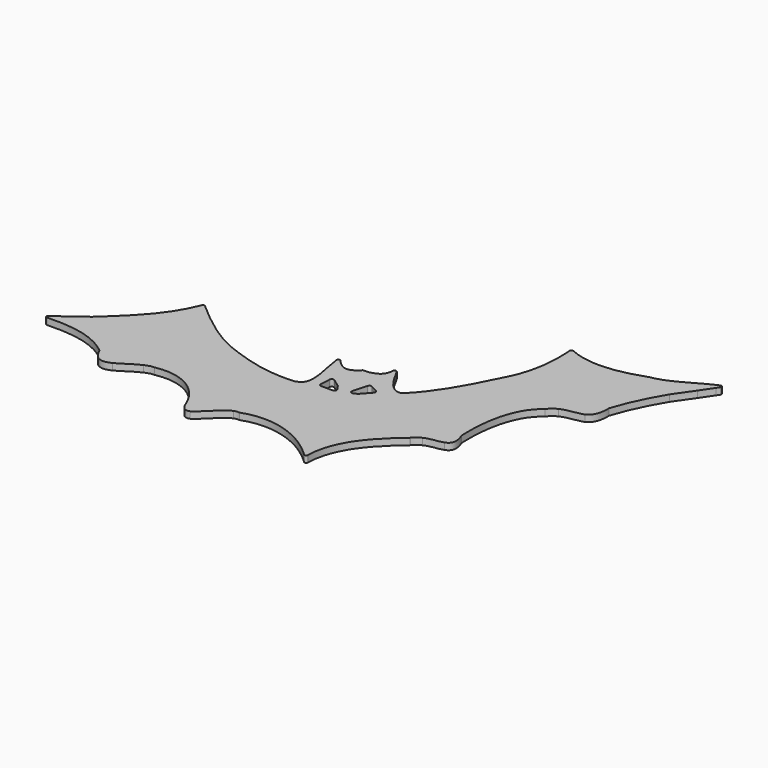
from build123d import *

# Parameters (mm, degrees)
F1_DEPTH    = 1.2
F2_R        = 0.3
F3_T1_DEPTH = 1.2
F4_R        = 0.4


# Not quite as in the source:
# - a fillet or chamfer that OpenCascade refuses, or shapes differently, is made with other operations: its cross-section is extruded or revolved along the edge and cut away or added


with BuildPart() as f1:
    # F0 (on Top) → F1 (new body)
    with BuildSketch(Plane.XY):
        with BuildLine():
            add(Edge.make_bspline(
                [(-38.4798780204, -12.2663156816), (-39.544490026, -13.1099494205), (-40.6234752996, -13.9226719378), (-41.7197013285, -14.6909028127)],
                knots=[0, 0, 0, 0, 0.5352911652, 0.5352911652, 0.5352911652, 0.5352911652], degree=3))
            add(Edge.make_bspline(
                [(-41.7197013286, -14.6909028123), (-38.0795273857, -14.7004525366), (-34.4057833476, -15.3318172874), (-31.2715117029, -17.7636174939)],
                knots=[0.2133521121, 0.2133521121, 0.2133521121, 0.2133521121, 1, 1, 1, 1], degree=3))
            add(Edge.make_bspline(
                [(-31.2715117029, -17.7636174939), (-29.0153017657, -22.7858694917), (-25.5082486685, -17.0450166263), (-22.2937322686, -17.0941546532)],
                knots=[0, 0, 0, 0, 1, 1, 1, 1], degree=3))
            add(Edge.make_bspline(
                [(-22.2937322686, -17.0941546532), (-18.3303199267, -16.3920818703), (-14.1754137574, -17.8912452003), (-12.0371793955, -22.4632093461)],
                knots=[0, 0, 0, 0, 1, 1, 1, 1], degree=3))
            add(Edge.make_bspline(
                [(-12.0371793955, -22.4632093461), (-10.273242702, -27.2684784847), (-7.0541938207, -19.6953683351), (-4.1345165041, -20.0729846223)],
                knots=[0, 0, 0, 0, 1, 1, 1, 1], degree=3))
            add(Edge.make_bspline(
                [(-4.1345165041, -20.0729846223), (1.2434419273, -18.2527364634), (7.1570299201, -20.3861330581), (11.4834791975, -24.5899863856)],
                knots=[0, 0, 0, 0, 1, 1, 1, 1], degree=3))
            add(Edge.make_bspline(
                [(11.4834791975, -24.5899863856), (11.3410479857, -18.4819489611), (15.805950917, -14.5268131434), (19.4643467655, -11.5875236785)],
                knots=[0, 0, 0, 0, 1, 1, 1, 1], degree=3))
            add(Edge.make_bspline(
                [(19.4643467655, -11.5875236785), (20.8953696781, -9.465229862), (24.9063475432, -10.9951342488), (24.8114189767, -8.5803924237)],
                knots=[0, 0, 0, 0, 0.8539890071, 0.8539890071, 0.8539890071, 0.8539890071], degree=3))
            add(Edge.make_bspline(
                [(24.8114189767, -8.5803924237), (24.7715269271, -8.4685484651), (24.7275843922, -8.3524176209), (24.6794406334, -8.2318174934)],
                knots=[0.9759440179, 0.9759440179, 0.9759440179, 0.9759440179, 1, 1, 1, 1], degree=3))
            add(Edge.make_bspline(
                [(24.6794406334, -8.2318174934), (24.6721729206, -8.0739743472), (24.6659042214, -7.915212537), (24.6606897414, -7.7556620666)],
                knots=[0, 0, 0, 0, 0.0312727725, 0.0312727725, 0.0312727725, 0.0312727725], degree=3))
            add(Edge.make_bspline(
                [(24.6606897414, -7.7556620666), (24.5901871692, -7.5161203522), (24.4939231594, -7.2512100585), (24.3692332397, -6.9579036653)],
                knots=[0.9371550745, 0.9371550745, 0.9371550745, 0.9371550745, 1, 1, 1, 1], degree=3))
            add(Edge.make_bspline(
                [(24.3692332397, -6.9579036653), (24.1388380843, -2.2591127335), (24.9211464491, 3.314156379), (28.5056438685, 5.8047525516)],
                knots=[0, 0, 0, 0, 1, 1, 1, 1], degree=3))
            add(Edge.make_bspline(
                [(28.5056438685, 5.8047525516), (30.9062919992, 8.9355748498), (35.8582398281, 5.7820329361), (35.6726384866, 11.4003236568)],
                knots=[0, 0, 0, 0, 1, 1, 1, 1], degree=3))
            add(Edge.make_bspline(
                [(35.6726384866, 11.4003236568), (36.7663971201, 14.6066645914), (38.3424158626, 17.4642666985), (40.1032277755, 20.1498568209)],
                knots=[0, 0, 0, 0, 0.5755878955, 0.5755878955, 0.5755878955, 0.5755878955], degree=3))
            add(Edge.make_bspline(
                [(40.1032277755, 20.1498568209), (41.2585835018, 22.0843550242), (42.5070626066, 23.9305479484), (43.7611872479, 25.743781902)],
                knots=[0.5268633096, 0.5268633096, 0.5268633096, 0.5268633096, 0.908526515, 0.908526515, 0.908526515, 0.908526515], degree=3))
            add(Edge.make_bspline(
                [(43.7611872479, 25.743781902), (40.5051598058, 24.6156248297), (37.6057351876, 22.1634385625), (34.1849912478, 21.6757304041)],
                knots=[0.0409615452, 0.0409615452, 0.0409615452, 0.0409615452, 1, 1, 1, 1], degree=3))
            add(Edge.make_bspline(
                [(34.1849912478, 21.6757304041), (29.819862337, 20.2040716593), (25.0759812483, 19.4382459028), (20.7234813058, 21.313829756)],
                knots=[0, 0, 0, 0, 0.9509269262, 0.9509269262, 0.9509269262, 0.9509269262], degree=3))
            add(Edge.make_bspline(
                [(20.7234813058, 21.313829756), (20.9800191175, 17.2558597069), (20.4243543566, 13.0954506221), (18.5978538652, 9.7460444081)],
                knots=[0.0959141779, 0.0959141779, 0.0959141779, 0.0959141779, 1, 1, 1, 1], degree=3))
            add(Edge.make_bspline(
                [(18.5978538652, 9.7460444081), (16.277791329, 4.965444658), (13.734376016, 0.0795420777), (10.2447861041, -3.272037287)],
                knots=[0, 0, 0, 0, 1, 1, 1, 1], degree=3))
            add(Edge.make_bspline(
                [(10.2447861041, -3.272037287), (10.1955990612, -3.2702979601), (10.1468874332, -3.2670014327), (10.0986391366, -3.2621927773)],
                knots=[0, 0, 0, 0, 0.0194783611, 0.0194783611, 0.0194783611, 0.0194783611], degree=3))
            add(Edge.make_bspline(
                [(10.0986391274, -3.2621927392), (10.0510770286, -3.3087890461), (10.0033383979, -3.3551002989), (9.9554213638, -3.4011222524)],
                knots=[0.9862685814, 0.9862685814, 0.9862685814, 0.9862685814, 1, 1, 1, 1], degree=3))
            add(Edge.make_bspline(
                [(9.9554213638, -3.4011222524), (7.6435278836, -3.319370212), (6.3819190636, 0.2025468295), (4.915882773, 2.4844337463)],
                knots=[0, 0, 0, 0, 0.9155241129, 0.9155241129, 0.9155241129, 0.9155241129], degree=3))
            add(Edge.make_bspline(
                [(4.915882772, 2.4844337459), (5.1701481527, 0.5226394908), (4.5999139224, -0.4439197046), (3.5342091981, -0.8428686021)],
                knots=[0.072121838, 0.072121838, 0.072121838, 0.072121838, 0.6923701781, 0.6923701781, 0.6923701781, 0.6923701781], degree=3))
            add(Edge.make_bspline(
                [(3.5342091981, -0.8428686021), (3.0006050925, -1.1239670726), (2.3072433966, -1.2205903145), (1.5090960129, -1.2041829107)],
                knots=[0.6335885985, 0.6335885985, 0.6335885985, 0.6335885985, 0.9752013666, 0.9752013666, 0.9752013666, 0.9752013666], degree=3))
            add(Edge.make_bspline(
                [(1.5090960151, -1.2041829145), (1.0819239999, -1.6929707802), (0.6747439774, -1.9863590245), (0.2827989549, -2.124205249)],
                knots=[0.0195076299, 0.0195076299, 0.0195076299, 0.0195076299, 0.2398921319, 0.2398921319, 0.2398921319, 0.2398921319], degree=3))
            add(Edge.make_bspline(
                [(0.2827989549, -2.124205249), (-1.0880546786, -2.8652191263), (-2.266017231, -1.6618946241), (-3.4430695093, -0.1227718969)],
                knots=[0.186179007, 0.186179007, 0.186179007, 0.186179007, 0.9421201193, 0.9421201193, 0.9421201193, 0.9421201193], degree=3))
            add(Edge.make_bspline(
                [(-3.4430695131, -0.1227718981), (-3.4255558663, -3.302165987), (-1.0028536904, -8.9139481262), (-3.5364033807, -9.7617317538)],
                knots=[0.0501467186, 0.0501467186, 0.0501467186, 0.0501467186, 0.9884755517, 0.9884755517, 0.9884755517, 0.9884755517], degree=3))
            add(Edge.make_bspline(
                [(-3.5364033807, -9.7617317538), (-3.6509693086, -9.8276644972), (-3.7789141725, -9.8807515971), (-3.9213733821, -9.9198831012)],
                knots=[0.949678724, 0.949678724, 0.949678724, 0.949678724, 1, 1, 1, 1], degree=3))
            add(Edge.make_bspline(
                [(-3.9213733821, -9.9198831012), (-8.6406616352, -10.3835421633), (-13.380489336, -8.9703992448), (-17.881091994, -7.1713692357)],
                knots=[0, 0, 0, 0, 1, 1, 1, 1], degree=3))
            add(Edge.make_bspline(
                [(-17.881091994, -7.1713692357), (-21.6865107135, -5.4322589935), (-25.1450968709, -2.5874337425), (-28.4908956865, 0.3476423008)],
                knots=[0, 0, 0, 0, 0.982318537, 0.982318537, 0.982318537, 0.982318537], degree=3))
            add(Edge.make_bspline(
                [(-28.4908956865, 0.3476423008), (-30.6388932539, -5.2082381627), (-34.7433771111, -8.8024351025), (-38.4798780204, -12.2663156816)],
                knots=[0.0168646563, 0.0168646563, 0.0168646563, 0.0168646563, 1, 1, 1, 1], degree=3))
        make_face()
        Polygon((1.7419457076, -7.1895932953), (2.7923465749, -8.7172033417), (-0.4901575656, -8.7172033417), (-0.3588544668, -5.6619801284), align=None, mode=Mode.SUBTRACT)
        Polygon((5.5462396091, -7.2971257007), (4.0783693834, -8.0565469849), (5.1914485132, -4.0645922322), (7.370299421, -5.2602795405), align=None, mode=Mode.SUBTRACT)
        with BuildLine():
            add(Edge.make_bspline(
                [(-41.7197013285, -14.6909028127), (-42.6335712737, -15.3313392638), (-43.559423096, -15.9408551794), (-44.4989181194, -16.511582528)],
                knots=[0.5352911652, 0.5352911652, 0.5352911652, 0.5352911652, 0.9815371902, 0.9815371902, 0.9815371902, 0.9815371902], degree=3))
            add(Edge.make_bspline(
                [(-44.4989181275, -16.5115825034), (-39.9561544079, -16.1990223611), (-35.1263871422, -16.4287457235), (-31.1552008978, -19.7099196026)],
                knots=[0.0118832119, 0.0118832119, 0.0118832119, 0.0118832119, 1, 1, 1, 1], degree=3))
            add(Edge.make_bspline(
                [(-31.1552008978, -19.7099196026), (-30.1758999076, -22.0313326024), (-28.9629739841, -22.2119628364), (-27.6404651178, -21.6685669613)],
                knots=[0, 0, 0, 0, 0.4303094298, 0.4303094298, 0.4303094298, 0.4303094298], degree=3))
            add(Edge.make_bspline(
                [(-27.6404651178, -21.6685669613), (-26.4136092273, -21.0807535834), (-25.1021498938, -19.9703779599), (-23.8017680882, -19.4302696749)],
                knots=[0.4615109586, 0.4615109586, 0.4615109586, 0.4615109586, 0.8561499184, 0.8561499184, 0.8561499184, 0.8561499184], degree=3))
            add(Edge.make_bspline(
                [(-23.8017680882, -19.4302696749), (-23.2308687956, -19.1588967961), (-22.6607361116, -18.9816611178), (-22.0994456213, -18.9907986567)],
                knots=[0.8268924715, 0.8268924715, 0.8268924715, 0.8268924715, 1, 1, 1, 1], degree=3))
            add(Edge.make_bspline(
                [(-22.0994456213, -18.9907986567), (-18.1016108647, -18.236655646), (-13.9106180306, -19.8470085712), (-11.7538116767, -24.7580792951)],
                knots=[0, 0, 0, 0, 1, 1, 1, 1], degree=3))
            add(Edge.make_bspline(
                [(-11.7538116767, -24.7580792951), (-11.2148278891, -26.3216901636), (-10.5411564558, -26.6651547457), (-9.7819920599, -26.395493941)],
                knots=[0, 0, 0, 0, 0.3029265659, 0.3029265659, 0.3029265659, 0.3029265659], degree=3))
            add(Edge.make_bspline(
                [(-9.7819920599, -26.395493941), (-8.3541917148, -25.6378360556), (-6.6604600485, -23.0798193477), (-5.0027480113, -22.4472612622)],
                knots=[0.340891627, 0.340891627, 0.340891627, 0.340891627, 0.895530138, 0.895530138, 0.895530138, 0.895530138], degree=3))
            add(Edge.make_bspline(
                [(-5.0027480113, -22.4472612622), (-4.5933732749, -22.2392803561), (-4.1851205843, -22.1351197775), (-3.7825114669, -22.1905713602)],
                knots=[0.8632922845, 0.8632922845, 0.8632922845, 0.8632922845, 1, 1, 1, 1], degree=3))
            add(Edge.make_bspline(
                [(-3.7825114669, -22.1905713602), (1.5220540535, -20.2786027831), (7.3432416965, -22.4275523556), (11.6789399787, -26.7459622382)],
                knots=[0, 0, 0, 0, 0.977859807, 0.977859807, 0.977859807, 0.977859807], degree=3))
            add(Edge.make_bspline(
                [(11.6789399765, -26.7459622393), (11.7340343899, -20.4259288614), (16.1222114441, -16.293306437), (19.7319529949, -13.2048206876)],
                knots=[0.021795606, 0.021795606, 0.021795606, 0.021795606, 1, 1, 1, 1], degree=3))
            add(Edge.make_bspline(
                [(19.7319529949, -13.2048206876), (20.0648448741, -12.6790700459), (20.5361472499, -12.361974633), (21.063139265, -12.1534402923)],
                knots=[0, 0, 0, 0, 0.1969486194, 0.1969486194, 0.1969486194, 0.1969486194], degree=3))
            add(Edge.make_bspline(
                [(21.063139265, -12.1534402923), (22.124821272, -11.6204399525), (23.5032142124, -11.6539154252), (24.4216825116, -11.314118977)],
                knots=[0.160105494, 0.160105494, 0.160105494, 0.160105494, 0.5755889685, 0.5755889685, 0.5755889685, 0.5755889685], degree=3))
            add(Edge.make_bspline(
                [(24.4216825116, -11.314118977), (25.1084151933, -10.9436420426), (25.3984004293, -10.2260920005), (24.8114189767, -8.5803924237)],
                knots=[0.6219783681, 0.6219783681, 0.6219783681, 0.6219783681, 0.9759440179, 0.9759440179, 0.9759440179, 0.9759440179], degree=3))
            add(Edge.make_bspline(
                [(19.4643467655, -11.5875236785), (20.8953696781, -9.465229862), (24.9063475432, -10.9951342488), (24.8114189767, -8.5803924237)],
                knots=[0, 0, 0, 0, 0.8539890071, 0.8539890071, 0.8539890071, 0.8539890071], degree=3))
            add(Edge.make_bspline(
                [(11.4834791975, -24.5899863856), (11.3410479857, -18.4819489611), (15.805950917, -14.5268131434), (19.4643467655, -11.5875236785)],
                knots=[0, 0, 0, 0, 1, 1, 1, 1], degree=3))
            add(Edge.make_bspline(
                [(-4.1345165041, -20.0729846223), (1.2434419273, -18.2527364634), (7.1570299201, -20.3861330581), (11.4834791975, -24.5899863856)],
                knots=[0, 0, 0, 0, 1, 1, 1, 1], degree=3))
            add(Edge.make_bspline(
                [(-12.0371793955, -22.4632093461), (-10.273242702, -27.2684784847), (-7.0541938207, -19.6953683351), (-4.1345165041, -20.0729846223)],
                knots=[0, 0, 0, 0, 1, 1, 1, 1], degree=3))
            add(Edge.make_bspline(
                [(-22.2937322686, -17.0941546532), (-18.3303199267, -16.3920818703), (-14.1754137574, -17.8912452003), (-12.0371793955, -22.4632093461)],
                knots=[0, 0, 0, 0, 1, 1, 1, 1], degree=3))
            add(Edge.make_bspline(
                [(-31.2715117029, -17.7636174939), (-29.0153017657, -22.7858694917), (-25.5082486685, -17.0450166263), (-22.2937322686, -17.0941546532)],
                knots=[0, 0, 0, 0, 1, 1, 1, 1], degree=3))
            add(Edge.make_bspline(
                [(-41.7197013286, -14.6909028123), (-38.0795273857, -14.7004525366), (-34.4057833476, -15.3318172874), (-31.2715117029, -17.7636174939)],
                knots=[0.2133521121, 0.2133521121, 0.2133521121, 0.2133521121, 1, 1, 1, 1], degree=3))
        make_face()
        with BuildLine():
            add(Edge.make_bspline(
                [(24.8114189767, -8.5803924237), (24.8021743196, -8.3452318072), (24.7539895843, -8.0726604911), (24.6606897414, -7.7556620666)],
                knots=[0.8539890071, 0.8539890071, 0.8539890071, 0.8539890071, 0.9371550745, 0.9371550745, 0.9371550745, 0.9371550745], degree=3))
            add(Edge.make_bspline(
                [(24.4216825116, -11.314118977), (25.1084151933, -10.9436420426), (25.3984004293, -10.2260920005), (24.8114189767, -8.5803924237)],
                knots=[0.6219783681, 0.6219783681, 0.6219783681, 0.6219783681, 0.9759440179, 0.9759440179, 0.9759440179, 0.9759440179], degree=3))
            add(Edge.make_bspline(
                [(24.4216825116, -11.314118977), (25.3598860798, -10.9670212705), (25.8181877184, -10.2304382024), (24.9688053737, -8.1027335681)],
                knots=[0.5755889685, 0.5755889685, 0.5755889685, 0.5755889685, 1, 1, 1, 1], degree=3))
            add(Edge.make_bspline(
                [(24.9688053737, -8.1027335681), (24.7364079173, -3.0554299243), (25.5255111036, 2.9312150112), (29.1411414432, 5.6065413944)],
                knots=[0, 0, 0, 0, 1, 1, 1, 1], degree=3))
            add(Edge.make_bspline(
                [(29.1411414432, 5.6065413944), (29.5613508158, 6.1901386685), (30.0590563565, 6.5704545189), (30.5937294572, 6.8320038295)],
                knots=[0, 0, 0, 0, 0.1735327764, 0.1735327764, 0.1735327764, 0.1735327764], degree=3))
            add(Edge.make_bspline(
                [(28.8517767028, 5.4774574692), (29.3469280526, 6.1651356964), (29.9496822108, 6.5705589099), (30.5937294572, 6.8320038295)],
                knots=[0, 0, 0, 0, 0.2044812389, 0.2044812389, 0.2044812389, 0.2044812389], degree=3))
            add(Edge.make_bspline(
                [(24.6606897414, -7.7556620666), (24.4991623707, -2.8133153423), (25.3492171484, 2.8857949517), (28.8517767028, 5.4774574692)],
                knots=[0.0312727725, 0.0312727725, 0.0312727725, 0.0312727725, 1, 1, 1, 1], degree=3))
        make_face()
        with BuildLine():
            add(Edge.make_bspline(
                [(24.6606897414, -7.7556620666), (24.5901871692, -7.5161203522), (24.4939231594, -7.2512100585), (24.3692332397, -6.9579036653)],
                knots=[0.9371550745, 0.9371550745, 0.9371550745, 0.9371550745, 1, 1, 1, 1], degree=3))
            add(Edge.make_bspline(
                [(24.6606897414, -7.7556620666), (24.4991623707, -2.8133153423), (25.3492171484, 2.8857949517), (28.8517767028, 5.4774574692)],
                knots=[0.0312727725, 0.0312727725, 0.0312727725, 0.0312727725, 1, 1, 1, 1], degree=3))
            add(Edge.make_bspline(
                [(28.8517767028, 5.4774574692), (29.3469280526, 6.1651356964), (29.9496822108, 6.5705589099), (30.5937294572, 6.8320038295)],
                knots=[0, 0, 0, 0, 0.2044812389, 0.2044812389, 0.2044812389, 0.2044812389], degree=3))
            add(Edge.make_bspline(
                [(30.5937294572, 6.8320038295), (31.899558591, 7.4707842529), (33.4258919031, 7.4011457737), (34.582316623, 7.8542845546)],
                knots=[0.1735327764, 0.1735327764, 0.1735327764, 0.1735327764, 0.5973509091, 0.5973509091, 0.5973509091, 0.5973509091], degree=3))
            add(Edge.make_bspline(
                [(34.582316623, 7.8542845546), (35.5230078327, 8.3313139642), (36.149586686, 9.2777125941), (36.0810189587, 11.4880572058)],
                knots=[0.6337459821, 0.6337459821, 0.6337459821, 0.6337459821, 1, 1, 1, 1], degree=3))
            add(Edge.make_bspline(
                [(36.0810189587, 11.4880572058), (37.0908856965, 14.6406619291), (38.5083280495, 17.4793973386), (40.1032277755, 20.1498568209)],
                knots=[0, 0, 0, 0, 0.5268633096, 0.5268633096, 0.5268633096, 0.5268633096], degree=3))
            add(Edge.make_bspline(
                [(35.6726384866, 11.4003236568), (36.7663971201, 14.6066645914), (38.3424158626, 17.4642666985), (40.1032277755, 20.1498568209)],
                knots=[0, 0, 0, 0, 0.5755878955, 0.5755878955, 0.5755878955, 0.5755878955], degree=3))
            add(Edge.make_bspline(
                [(28.5056438685, 5.8047525516), (30.9062919992, 8.9355748498), (35.8582398281, 5.7820329361), (35.6726384866, 11.4003236568)],
                knots=[0, 0, 0, 0, 1, 1, 1, 1], degree=3))
            add(Edge.make_bspline(
                [(24.3692332397, -6.9579036653), (24.1388380843, -2.2591127335), (24.9211464491, 3.314156379), (28.5056438685, 5.8047525516)],
                knots=[0, 0, 0, 0, 1, 1, 1, 1], degree=3))
        make_face()
        with BuildLine():
            add(Edge.make_bspline(
                [(43.7611872479, 25.743781902), (40.5051598058, 24.6156248297), (37.6057351876, 22.1634385625), (34.1849912478, 21.6757304041)],
                knots=[0.0409615452, 0.0409615452, 0.0409615452, 0.0409615452, 1, 1, 1, 1], degree=3))
            add(Edge.make_bspline(
                [(43.7611872479, 25.743781902), (44.0617641701, 26.1783609406), (44.3626653834, 26.6110467488), (44.6626865653, 27.0426012886)],
                knots=[0.908526515, 0.908526515, 0.908526515, 0.908526515, 1, 1, 1, 1], degree=3))
            add(Edge.make_bspline(
                [(44.6626865653, 27.0426012886), (44.2714142278, 26.9147311358), (43.8856744157, 26.7649674364), (43.504013168, 26.5991099509)],
                knots=[0, 0, 0, 0, 0.1131398608, 0.1131398608, 0.1131398608, 0.1131398608], degree=3))
            add(Edge.make_bspline(
                [(43.504013168, 26.5991099509), (41.4906521544, 25.678347586), (39.5816149567, 24.3463766166), (37.5601123101, 23.4679563812)],
                knots=[0.1418082406, 0.1418082406, 0.1418082406, 0.1418082406, 0.7417521523, 0.7417521523, 0.7417521523, 0.7417521523], degree=3))
            add(Edge.make_bspline(
                [(37.5601123101, 23.4679563812), (36.5981547538, 23.028007783), (35.6128416392, 22.6823510278), (34.5804529778, 22.525603686)],
                knots=[0.7130522103, 0.7130522103, 0.7130522103, 0.7130522103, 1, 1, 1, 1], degree=3))
            add(Edge.make_bspline(
                [(34.5804529778, 22.525603686), (30.0575614605, 20.9017602032), (25.1315516694, 20.077941371), (20.6444141255, 22.3077248958)],
                knots=[0, 0, 0, 0, 0.9768105292, 0.9768105292, 0.9768105292, 0.9768105292], degree=3))
            add(Edge.make_bspline(
                [(20.6444141255, 22.3077248958), (20.6760436931, 21.9774467695), (20.7024832551, 21.645981418), (20.7234813058, 21.313829756)],
                knots=[0.0219132354, 0.0219132354, 0.0219132354, 0.0219132354, 0.0959141779, 0.0959141779, 0.0959141779, 0.0959141779], degree=3))
            add(Edge.make_bspline(
                [(34.1849912478, 21.6757304041), (29.819862337, 20.2040716593), (25.0759812483, 19.4382459028), (20.7234813058, 21.313829756)],
                knots=[0, 0, 0, 0, 0.9509269262, 0.9509269262, 0.9509269262, 0.9509269262], degree=3))
        make_face()
        with BuildLine():
            add(Edge.make_bspline(
                [(43.7611872479, 25.743781902), (44.0617641701, 26.1783609406), (44.3626653834, 26.6110467488), (44.6626865653, 27.0426012886)],
                knots=[0.908526515, 0.908526515, 0.908526515, 0.908526515, 1, 1, 1, 1], degree=3))
            add(Edge.make_bspline(
                [(44.0214882714, 25.83083868), (43.9344585538, 25.8027955289), (43.8476970346, 25.7737560436), (43.7611872479, 25.743781902)],
                knots=[0.0154807366, 0.0154807366, 0.0154807366, 0.0154807366, 0.0409615452, 0.0409615452, 0.0409615452, 0.0409615452], degree=3))
            add(Edge.make_bspline(
                [(44.0214882714, 25.83083868), (44.3317305912, 26.2795519358), (44.6423597936, 26.7262217799), (44.9520513056, 27.171686254)],
                knots=[0.9055781271, 0.9055781271, 0.9055781271, 0.9055781271, 1, 1, 1, 1], degree=3))
            add(Edge.make_bspline(
                [(44.9520513056, 27.171686254), (44.4616346972, 27.0114152295), (43.9799096269, 26.816749781), (43.504013168, 26.5991099509)],
                knots=[0, 0, 0, 0, 0.1418082406, 0.1418082406, 0.1418082406, 0.1418082406], degree=3))
            add(Edge.make_bspline(
                [(44.6626865653, 27.0426012886), (44.2714142278, 26.9147311358), (43.8856744157, 26.7649674364), (43.504013168, 26.5991099509)],
                knots=[0, 0, 0, 0, 0.1131398608, 0.1131398608, 0.1131398608, 0.1131398608], degree=3))
        make_face()
        with BuildLine():
            add(Edge.make_bspline(
                [(40.1032277755, 20.1498568209), (41.2585835018, 22.0843550242), (42.5070626066, 23.9305479484), (43.7611872479, 25.743781902)],
                knots=[0.5268633096, 0.5268633096, 0.5268633096, 0.5268633096, 0.908526515, 0.908526515, 0.908526515, 0.908526515], degree=3))
            add(Edge.make_bspline(
                [(40.1032277755, 20.1498568209), (40.8750605545, 21.3270560846), (41.6823997153, 22.4712047589), (42.5001916972, 23.5971873103)],
                knots=[0.5755878955, 0.5755878955, 0.5755878955, 0.5755878955, 0.8278905984, 0.8278905984, 0.8278905984, 0.8278905984], degree=3))
            add(Edge.make_bspline(
                [(42.5001916972, 23.5971873103), (43.0023193892, 24.3497455182), (43.511380868, 25.0930542478), (44.0214882714, 25.83083868)],
                knots=[0.750327559, 0.750327559, 0.750327559, 0.750327559, 0.9055781271, 0.9055781271, 0.9055781271, 0.9055781271], degree=3))
            add(Edge.make_bspline(
                [(44.0214882714, 25.83083868), (43.9344585538, 25.8027955289), (43.8476970346, 25.7737560436), (43.7611872479, 25.743781902)],
                knots=[0.0154807366, 0.0154807366, 0.0154807366, 0.0154807366, 0.0409615452, 0.0409615452, 0.0409615452, 0.0409615452], degree=3))
        make_face()
        with BuildLine():
            add(Edge.make_bspline(
                [(-44.5870734222, -16.5177178863), (-44.5577005497, -16.5156505029), (-44.528315348, -16.5136051487), (-44.4989181275, -16.5115825034)],
                knots=[0.0054888914, 0.0054888914, 0.0054888914, 0.0054888914, 0.0118832119, 0.0118832119, 0.0118832119, 0.0118832119], degree=3))
            add(Edge.make_bspline(
                [(-44.5870734245, -16.5177178787), (-44.6540732421, -16.5588967025), (-44.721142128, -16.599880307), (-44.7882806885, -16.6406658208)],
                knots=[0.9496472025, 0.9496472025, 0.9496472025, 0.9496472025, 0.981537011, 0.981537011, 0.981537011, 0.981537011], degree=3))
            add(Edge.make_bspline(
                [(-44.7882806966, -16.6406657962), (-40.245516975, -16.3281058214), (-35.4157514066, -16.5578295219), (-31.4445656382, -19.8390030077)],
                knots=[0.0118833303, 0.0118833303, 0.0118833303, 0.0118833303, 1, 1, 1, 1], degree=3))
            add(Edge.make_bspline(
                [(-31.4445656382, -19.8390030077), (-30.3942560066, -22.3287405419), (-29.0752130664, -22.3559859521), (-27.6404651178, -21.6685669613)],
                knots=[0, 0, 0, 0, 0.4615109586, 0.4615109586, 0.4615109586, 0.4615109586], degree=3))
            add(Edge.make_bspline(
                [(-31.1552008978, -19.7099196026), (-30.1758999076, -22.0313326024), (-28.9629739841, -22.2119628364), (-27.6404651178, -21.6685669613)],
                knots=[0, 0, 0, 0, 0.4303094298, 0.4303094298, 0.4303094298, 0.4303094298], degree=3))
            add(Edge.make_bspline(
                [(-44.4989181275, -16.5115825034), (-39.9561544079, -16.1990223611), (-35.1263871422, -16.4287457235), (-31.1552008978, -19.7099196026)],
                knots=[0.0118832119, 0.0118832119, 0.0118832119, 0.0118832119, 1, 1, 1, 1], degree=3))
        make_face()
        with BuildLine():
            add(Edge.make_bspline(
                [(-41.8254731926, -14.6907992634), (-42.7336947269, -15.3324841221), (-43.6536816895, -15.9440450669), (-44.5870734245, -16.5177178787)],
                knots=[0.5053820577, 0.5053820577, 0.5053820577, 0.5053820577, 0.9496472025, 0.9496472025, 0.9496472025, 0.9496472025], degree=3))
            add(Edge.make_bspline(
                [(-44.5870734222, -16.5177178863), (-44.5577005497, -16.5156505029), (-44.528315348, -16.5136051487), (-44.4989181275, -16.5115825034)],
                knots=[0.0054888914, 0.0054888914, 0.0054888914, 0.0054888914, 0.0118832119, 0.0118832119, 0.0118832119, 0.0118832119], degree=3))
            add(Edge.make_bspline(
                [(-41.7197013285, -14.6909028127), (-42.6335712737, -15.3313392638), (-43.559423096, -15.9408551794), (-44.4989181194, -16.511582528)],
                knots=[0.5352911652, 0.5352911652, 0.5352911652, 0.5352911652, 0.9815371902, 0.9815371902, 0.9815371902, 0.9815371902], degree=3))
            add(Edge.make_bspline(
                [(-41.8254731929, -14.6907992625), (-41.7902194019, -14.6907761492), (-41.7549619402, -14.6908103087), (-41.7197013286, -14.6909028123)],
                knots=[0.205732233, 0.205732233, 0.205732233, 0.205732233, 0.2133521121, 0.2133521121, 0.2133521121, 0.2133521121], degree=3))
        make_face()
        with BuildLine():
            add(Edge.make_bspline(
                [(-38.7692427608, -12.3954006471), (-39.7743698771, -13.1918960134), (-40.7923089368, -13.9608387477), (-41.8254731926, -14.6907992634)],
                knots=[0, 0, 0, 0, 0.5053820577, 0.5053820577, 0.5053820577, 0.5053820577], degree=3))
            add(Edge.make_bspline(
                [(-41.8254731929, -14.6907992625), (-41.7902194019, -14.6907761492), (-41.7549619402, -14.6908103087), (-41.7197013286, -14.6909028123)],
                knots=[0.205732233, 0.205732233, 0.205732233, 0.205732233, 0.2133521121, 0.2133521121, 0.2133521121, 0.2133521121], degree=3))
            add(Edge.make_bspline(
                [(-38.4798780204, -12.2663156816), (-39.544490026, -13.1099494205), (-40.6234752996, -13.9226719378), (-41.7197013285, -14.6909028127)],
                knots=[0, 0, 0, 0, 0.5352911652, 0.5352911652, 0.5352911652, 0.5352911652], degree=3))
            add(Edge.make_bspline(
                [(-28.4908956865, 0.3476423008), (-30.6388932539, -5.2082381627), (-34.7433771111, -8.8024351025), (-38.4798780204, -12.2663156816)],
                knots=[0.0168646563, 0.0168646563, 0.0168646563, 0.0168646563, 1, 1, 1, 1], degree=3))
            add(Edge.make_bspline(
                [(-28.4908956865, 0.3476423008), (-28.5511191431, 0.4004728607), (-28.6113060578, 0.453332661), (-28.6714577954, 0.5062157798)],
                knots=[0.982318537, 0.982318537, 0.982318537, 0.982318537, 1, 1, 1, 1], degree=3))
            add(Edge.make_bspline(
                [(-28.6714577954, 0.5062157798), (-30.7873334761, -5.2139738594), (-34.9686460951, -8.8720992673), (-38.7692427608, -12.3954006471)],
                knots=[0, 0, 0, 0, 1, 1, 1, 1], degree=3))
        make_face()
        with BuildLine():
            add(Edge.make_bspline(
                [(24.8114189767, -8.5803924237), (24.7715269271, -8.4685484651), (24.7275843922, -8.3524176209), (24.6794406334, -8.2318174934)],
                knots=[0.9759440179, 0.9759440179, 0.9759440179, 0.9759440179, 1, 1, 1, 1], degree=3))
            add(Edge.make_bspline(
                [(24.8114189767, -8.5803924237), (24.8021743196, -8.3452318072), (24.7539895843, -8.0726604911), (24.6606897414, -7.7556620666)],
                knots=[0.8539890071, 0.8539890071, 0.8539890071, 0.8539890071, 0.9371550745, 0.9371550745, 0.9371550745, 0.9371550745], degree=3))
            add(Edge.make_bspline(
                [(24.6794406334, -8.2318174934), (24.6721729206, -8.0739743472), (24.6659042214, -7.915212537), (24.6606897414, -7.7556620666)],
                knots=[0, 0, 0, 0, 0.0312727725, 0.0312727725, 0.0312727725, 0.0312727725], degree=3))
        make_face()
        with BuildLine():
            add(Edge.make_bspline(
                [(-5.0027480113, -22.4472612622), (-4.5933732749, -22.2392803561), (-4.1851205843, -22.1351197775), (-3.7825114669, -22.1905713602)],
                knots=[0.8632922845, 0.8632922845, 0.8632922845, 0.8632922845, 1, 1, 1, 1], degree=3))
            add(Edge.make_bspline(
                [(-5.0027480113, -22.4472612622), (-4.6905068951, -22.3281147288), (-4.3795436918, -22.2772800678), (-4.0718762073, -22.3196552855)],
                knots=[0.895530138, 0.895530138, 0.895530138, 0.895530138, 1, 1, 1, 1], degree=3))
            add(Edge.make_bspline(
                [(-4.0718762073, -22.3196552855), (1.352792526, -20.3643969105), (7.3177424001, -22.6560283326), (11.6817673263, -27.171687254)],
                knots=[0, 0, 0, 0, 1, 1, 1, 1], degree=3))
            add(Edge.make_bspline(
                [(11.6817673263, -27.171687254), (11.6786360074, -27.0286845368), (11.6777124047, -26.886780414), (11.6789399765, -26.7459622393)],
                knots=[0, 0, 0, 0, 0.021795606, 0.021795606, 0.021795606, 0.021795606], degree=3))
            add(Edge.make_bspline(
                [(-3.7825114669, -22.1905713602), (1.5220540535, -20.2786027831), (7.3432416965, -22.4275523556), (11.6789399787, -26.7459622382)],
                knots=[0, 0, 0, 0, 0.977859807, 0.977859807, 0.977859807, 0.977859807], degree=3))
        make_face()
    extrude(amount=F1_DEPTH)

    # F2
    f2_edges = [f1.edges().sort_by_distance(p)[0] for p in [
        (-28.671458, 0.506216, 0.6),
        (20.644414, 22.307725, 0.6),
        (-3.44307, -0.122772, 0.6),
        (4.915883, 2.484434, 0.6),
        (44.952051, 27.171686, 0.6),
        (-44.788281, -16.640666, 0.6),
        (11.681767, -27.171687, 0.6),
        (19.731953, -13.204821, 0.6),
    ]]
    fillet(f2_edges, radius=F2_R)

    # F3: fillet of radius 1 on 2 edges, made by hand

    # F3_s2 → F3_t1 (join)
    with BuildSketch(Plane.XY):
        with BuildLine():
            ThreePointArc((10.098639132, -3.2621927582), (9.7578871461, -3.3500201076), (9.4078087441, -3.3143736255))
            Line((9.4078087441, -3.3143736255), (9.4023135559, -3.3336038857))
            ThreePointArc((9.4023135559, -3.3336038857), (9.6758319606, -3.3942228207), (9.9547145753, -3.4211097598))
            Line((9.9547145753, -3.4211097598), (9.9692753838, -3.4155467499))
            ThreePointArc((9.9692753838, -3.4155467499), (10.041128116, -3.3461902864), (10.1069605515, -3.2803794011))
            Line((10.1069605515, -3.2803794011), (10.098639132, -3.2621927582))
        make_face()
        with BuildLine():
            ThreePointArc((10.5063632487, -3.0162040136), (10.3173567223, -3.1638212956), (10.098639132, -3.2621927582))
            Line((10.098639132, -3.2621927582), (10.1045964886, -3.2812849006))
            ThreePointArc((10.1045964886, -3.2812849006), (10.170290563, -3.2882392807), (10.2440793161, -3.2920247944))
            Line((10.2440793161, -3.2920247944), (10.2586401241, -3.2864617846))
            ThreePointArc((10.2586401241, -3.2864617846), (10.39013597, -3.1590080543), (10.5204750877, -3.0303763811))
            Line((10.5204750877, -3.0303763811), (10.5063632487, -3.0162040136))
        make_face()
    extrude(amount=F3_T1_DEPTH)

    # F4
    f4_edges = [f1.edges().sort_by_distance(p)[0] for p in [
        (7.370299, -5.26028, 0.6),
        (5.191449, -4.064592, 0.6),
        (4.078369, -8.056547, 0.6),
        (-0.490158, -8.717203, 0.6),
        (2.792347, -8.717203, 0.6),
        (-0.358854, -5.66198, 0.6),
        (5.54624, -7.297126, 0.6),
        (1.741946, -7.189593, 0.6),
    ]]
    fillet(f4_edges, radius=F4_R)


solid = f1.part
